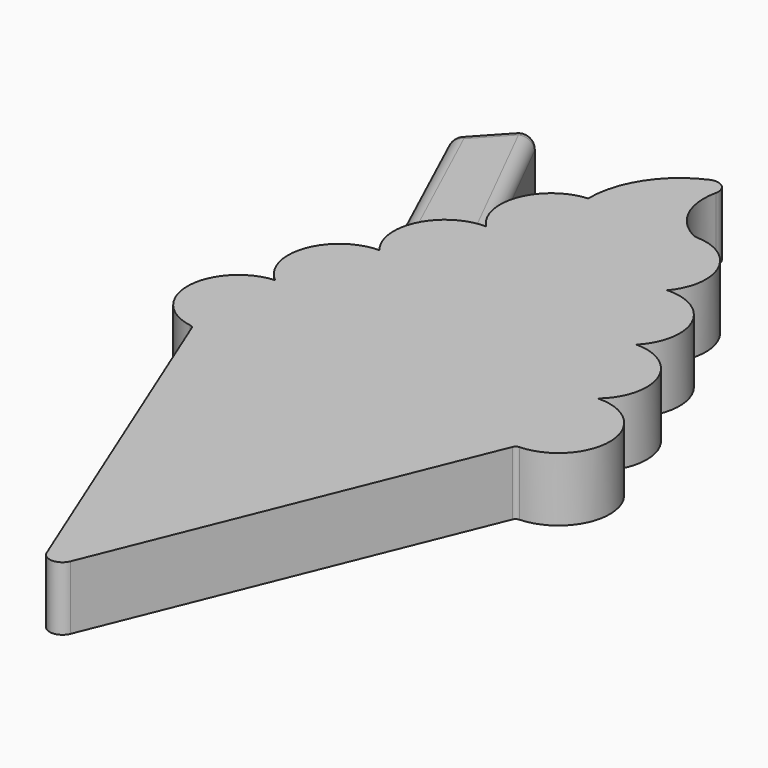
from build123d import *

# Parameters (mm, degrees)
F1_DEPTH     = 25
F2_R         = 5
F3_R         = 5
F4_R         = 2
F6_R         = 5
F7_DEPTH     = 20
F8_T1_DEPTH  = 16.879655815
F8_T3_DEPTH  = 23.3726224193
F8_T5_DEPTH  = 33.0268060681
F8_T10_DEPTH = 5.1
F8_T16_DEPTH = 5.1
F8_T22_DEPTH = 98.4210661838
F8_S23_R     = 20
F8_T24_DEPTH = 53
F8_S25_R     = 20
F8_T26_DEPTH = 53
F8_T30_DEPTH = 70.867251183
F8_S31_R     = 20
F8_T32_DEPTH = 39
F8_S33_R     = 20
F8_T34_DEPTH = 39


# Not quite as in the source:
# - a fillet or chamfer that OpenCascade refuses, or shapes differently, is made with other operations: its cross-section is extruded or revolved along the edge and cut away or added
# - two fillets or chamfers of one size are made in one step


with BuildPart() as f1:
    # F0 (on Top) → F1 (new body)
    with BuildSketch(Plane.XY):
        with BuildLine():
            ThreePointArc((-62.7989065684, 39.6886658546), (-81.243248627, 20.090620438), (-63.3367104763, 0))
            Line((-63.3367104763, 0), (0, -156.2183324342))
            Line((0, -156.2183324342), (63.3367104763, 0))
            ThreePointArc((63.3367104763, 0), (83.9060549488, 20.1553189736), (63.1791622356, 40.1485861756))
            ThreePointArc((63.1791622356, 40.1485861756), (68.8985621757, 62.3156526678), (50.0641206725, 75.3292680691))
            ThreePointArc((50.0641206725, 75.3292680691), (54.0847867027, 97.4676528526), (34.9687938538, 109.335788913))
            ThreePointArc((34.9687938538, 109.335788913), (37.8165399559, 130.8078112166), (19.4443891765, 142.2804515145))
            ThreePointArc((19.4443891765, 142.2804515145), (6.5496116272, 157.6455026462), (10.1508991793, 177.3784905672))
            ThreePointArc((10.1508991793, 177.3784905672), (-12.7726518652, 165.7418593556), (-21.8806297798, 141.7013702435))
            ThreePointArc((-21.8806297798, 141.7013702435), (-36.0248561638, 134.2091888045), (-40.144512278, 118.7424387834))
            Line((-40.144512278, 118.7424387834), (-34.6308081302, 107.732548238))
            ThreePointArc((-34.6308081302, 107.732548238), (-50.0933619749, 100.6048777691), (-54.4620472952, 84.1486070408))
            Line((-54.4620472952, 84.1486070408), (-50.2881059675, 75.0966394345))
            ThreePointArc((-50.2881059675, 75.0966394345), (-68.9068668709, 61.7610342158), (-62.7989065684, 39.6886658546))
        make_face()
        with BuildLine():
            Line((-19.4251702535, 141.7357782283), (-21.8806297798, 141.7013702435))
            ThreePointArc((-21.8806297798, 141.7013702435), (-20.6534286134, 141.7562965225), (-19.4251702535, 141.7357782283))
        make_face(mode=Mode.SUBTRACT)
        with BuildLine():
            ThreePointArc((-40.144512278, 118.7424387834), (-38.2560486822, 112.8026084286), (-34.6308081302, 107.732548238))
            Line((-34.6308081302, 107.732548238), (-40.144512278, 118.7424387834))
        make_face()
        with BuildLine():
            ThreePointArc((-54.4620472952, 84.1486070408), (-52.9480489841, 79.3584206811), (-50.2881059675, 75.0966394345))
            Line((-50.2881059675, 75.0966394345), (-54.4620472952, 84.1486070408))
        make_face()
        with BuildLine():
            ThreePointArc((-19.4251702535, 141.7357782283), (-20.6534286134, 141.7562965225), (-21.8806297798, 141.7013702435))
            Line((-21.8806297798, 141.7013702435), (-19.4251702535, 141.7357782283))
        make_face()
    extrude(amount=F1_DEPTH)

    # F2
    f2_edges = [f1.edges().sort_by_distance(p)[0] for p in [
        (10.150899, 177.378491, 12.5),
    ]]
    fillet(f2_edges, radius=F2_R)

    # F3
    f3_edges = [f1.edges().sort_by_distance(p)[0] for p in [
        (0, -156.218332, 12.5),
    ]]
    fillet(f3_edges, radius=F3_R)

    # F4
    f4_edges = [f1.edges().sort_by_distance(p)[0] for p in [
        (63.33671, 0, 12.5),
        (-63.33671, 0, 12.5),
    ]]
    fillet(f4_edges, radius=F4_R)

    # F6
    f6_edges = [f1.edges().sort_by_distance(p)[0] for p in [
        (19.444389, 142.280452, 12.5),
    ]]
    fillet(f6_edges, radius=F6_R)

    # F0 (on Top) → F7 (join)
    with BuildSketch(Plane.XY):
        with BuildLine():
            Line((-88.1787538528, 157.26955235), (-54.4620472952, 84.1486070408))
            ThreePointArc((-54.4620472952, 84.1486070408), (-50.0933619749, 100.6048777691), (-34.6308081302, 107.732548238))
            ThreePointArc((-34.6308081302, 107.732548238), (-38.2560486822, 112.8026084286), (-40.144512278, 118.7424387834))
            Line((-40.144512278, 118.7424387834), (-69.5091858506, 177.3784905672))
            Line((-69.5091858506, 177.3784905672), (-88.1787538528, 157.26955235))
        make_face()
    extrude(amount=F7_DEPTH)

    # F8: fillet of radius 5 on 5 edges, made by hand

    # F8_s2 → F8_t1 (cut)
    with BuildSketch(Plane(origin=(51.3609651153, 55.3207484048, 0), x_dir=(0, 0, 1), z_dir=(-0.6803920453, -0.7328483231, 0))):
        with BuildLine():
            ThreePointArc((20, 166.626604285), (18.5355339059, 170.1621381909), (15, 171.626604285))
            Line((15, 171.626604285), (20, 171.626604285))
            Line((20, 171.626604285), (20, 166.626604285))
        make_face()
    extrude(amount=F8_T1_DEPTH, mode=Mode.SUBTRACT)

    # F8_s4 → F8_t3 (cut)
    with BuildSketch(Plane.XY.offset(-8.3726224193)):
        with BuildLine():
            ThreePointArc((-85.9000875758, 159.72389727), (-87.1734696665, 157.1092566329), (-86.7763850028, 154.2282548314))
            Line((-86.7763850028, 154.2282548314), (-88.1787538528, 157.26955235))
            Line((-88.1787538528, 157.26955235), (-85.9000875758, 159.72389727))
        make_face()
    extrude(amount=F8_T3_DEPTH, mode=Mode.SUBTRACT)

    # F8_s6 → F8_t5 (cut)
    with BuildSketch(Plane.XY.offset(-18.0268060681)):
        with BuildLine():
            ThreePointArc((-66.280350029, 170.9310773526), (-70.0434123782, 173.6418343313), (-74.4153040312, 172.0941247282))
            Line((-74.4153040312, 172.0941247282), (-69.5091858506, 177.3784905672))
            Line((-69.5091858506, 177.3784905672), (-66.280350029, 170.9310773526))
        make_face()
    extrude(amount=F8_T5_DEPTH, mode=Mode.SUBTRACT)


with BuildPart() as f8_tool8:
    # F8_s9 → F8_t10 (new body)
    with BuildSketch(Plane.XY.offset(15)):
        Polygon((-82.2358459604, 156.3219370433), (-85.9733724081, 159.7919364745), (-88.2976120107, 157.2885046562), (-86.8671957836, 154.1863811872), align=None)
    extrude(amount=F8_T10_DEPTH)

    # F8_s11 → F8_t12 (revolve, cut)
    with BuildSketch(Plane(origin=(-82.2358459604, 156.3219370433, 15), x_dir=(0.9875247412, -0.1574639179, 0), z_dir=(-0.1574639179, -0.9875247412, 0))):
        with BuildLine():
            ThreePointArc((0, -5), (5, 0), (0, 5))
            Line((0, 5), (0, -5))
        make_face()
    revolve(axis=Axis((-82.2358459604, 156.3219370433, 15), (0, 0, 1)), mode=Mode.SUBTRACT)


with BuildPart() as f1_1:
    add(f1.part)

    # F8_t7: cut F8_tool8
    add(f8_tool8.part, mode=Mode.SUBTRACT)


with BuildPart() as f8_tool14:
    # F8_s15 → F8_t16 (new body)
    with BuildSketch(Plane.XY.offset(15)):
        Polygon((-70.7510624158, 168.6921645015), (-74.4885888636, 172.1621639327), (-69.4843483193, 177.5522170885), (-66.1909357813, 170.9758556096), align=None)
    extrude(amount=F8_T16_DEPTH)

    # F8_s17 → F8_t18 (revolve, cut)
    with BuildSketch(Plane(origin=(-70.7510624158, 168.6921645015, 15), x_dir=(-0.1415300075, -0.989933966, 0), z_dir=(-0.989933966, 0.1415300075, 0))):
        with BuildLine():
            ThreePointArc((0, -5), (5, 0), (0, 5))
            Line((0, 5), (0, -5))
        make_face()
    revolve(axis=Axis((-70.7510624158, 168.6921645015, 15), (0, 0, 1)), mode=Mode.SUBTRACT)


with BuildPart() as f1_2:
    add(f1_1.part)

    # F8_t13: cut F8_tool14
    add(f8_tool14.part, mode=Mode.SUBTRACT)


with BuildPart() as f8_tool20:
    # F8_s21 → F8_t22 (new body)
    with BuildSketch(Plane(origin=(-73.8618913818, 160.1832406418, 0), x_dir=(0, 0, 1), z_dir=(0.4187364424, -0.9081078085, 0))):
        with BuildLine():
            ThreePointArc((20, 9.2213220725), (18.5355339059, 12.7568559784), (15, 14.2213220725))
            Line((15, 14.2213220725), (20, 14.2213220725))
            Line((20, 14.2213220725), (20, 9.2213220725))
        make_face()
    extrude(amount=F8_T22_DEPTH)

    # F8_s23 → F8_t24 (cut, symmetric)
    with BuildSketch(Plane.XY.offset(17.5)):
        with Locations((-34.7858928144, 87.7331495285)):
            Circle(F8_S23_R)
    extrude(amount=F8_T24_DEPTH, both=True, mode=Mode.SUBTRACT)

    # F8_s25 → F8_t26 (cut, symmetric)
    with BuildSketch(Plane.XY.offset(17.5)):
        with Locations((-50.049379468, 55.0980642438)):
            Circle(F8_S25_R)
    extrude(amount=F8_T26_DEPTH, both=True, mode=Mode.SUBTRACT)


with BuildPart() as f1_3:
    add(f1_2.part)

    # F8_t19: cut F8_tool20
    add(f8_tool20.part, mode=Mode.SUBTRACT)


with BuildPart() as f8_tool28:
    # F8_s29 → F8_t30 (new body)
    with BuildSketch(Plane(origin=(-49.9943289817, 99.8298195219, 0), x_dir=(0, 0, 1), z_dir=(-0.4477825702, 0.8941424774, 0))):
        with BuildLine():
            ThreePointArc((15, 17.2758807713), (18.5355339059, 15.8114146772), (20, 12.2758807713))
            Line((20, 12.2758807713), (20, 17.2758807713))
            Line((20, 17.2758807713), (15, 17.2758807713))
        make_face()
    extrude(amount=F8_T30_DEPTH)

    # F8_s31 → F8_t32 (cut, symmetric)
    with BuildSketch(Plane.XY.offset(17.5)):
        with Locations((-20.3731991351, 121.7582598329)):
            Circle(F8_S31_R)
    extrude(amount=F8_T32_DEPTH, both=True, mode=Mode.SUBTRACT)

    # F8_s33 → F8_t34 (cut, symmetric)
    with BuildSketch(Plane.XY.offset(17.5)):
        with Locations((-34.7858928144, 87.7331495285)):
            Circle(F8_S33_R)
    extrude(amount=F8_T34_DEPTH, both=True, mode=Mode.SUBTRACT)


with BuildPart() as f1_4:
    add(f1_3.part)

    # F8_t27: cut F8_tool28
    add(f8_tool28.part, mode=Mode.SUBTRACT)


solid = f1_4.part
